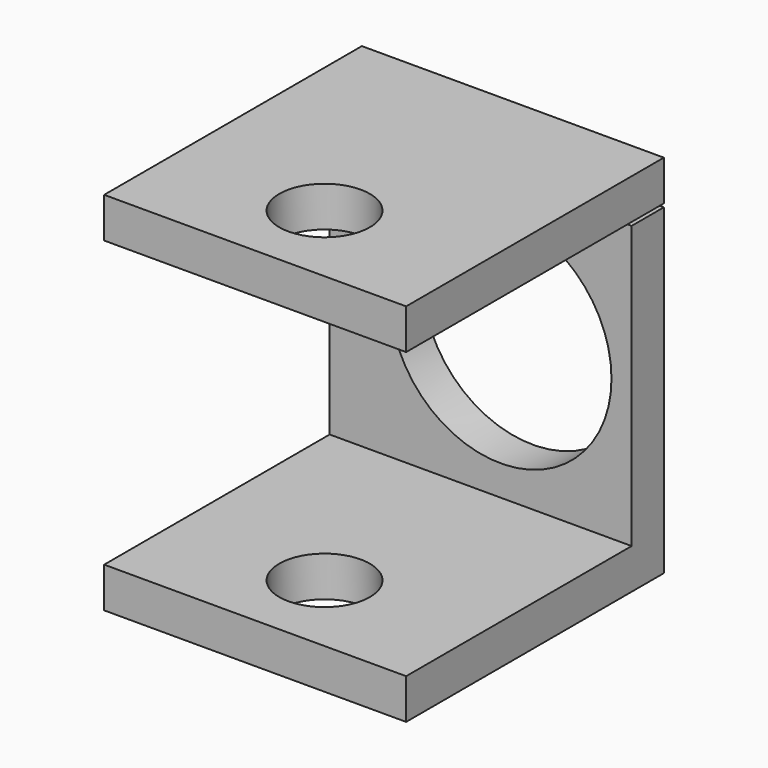
from build123d import *

# Parameters (mm, degrees)
F0_W     = 20.6375
F0_H     = 22.225
F0_R     = 8.73125
F1_DEPTH = 3.175
F2_DEPTH = 25.4
F4_D     = 7.14375


# Not quite as in the source:
# - a length typed as a fraction of an inch, garbled in the dataset ("3 / 203.2 mm" for 3/8 in), is restored


with BuildPart() as f1:
    # F0 (on Front) → F1 (new body)
    with BuildSketch(Plane.XZ):
        Rectangle(F0_W, F0_H)
        Circle(F0_R, mode=Mode.SUBTRACT)
        Polygon((-10.31875, -11.1125), (-10.31875, 11.1125), (-10.31875, 11.3854380324), (-13.49375, 11.3854380324), (-13.49375, -11.1125), align=None)
    extrude(amount=F1_DEPTH)

    # F0 (on Front) → F2 (join)
    with BuildSketch(Plane.XZ):
        Polygon((10.31875, -14.2875), (10.31875, -11.1125), (-10.31875, -11.1125), (-13.49375, -11.1125), (-13.49375, -14.2875), align=None)
        Polygon((-13.49375, 11.3854380324), (-10.31875, 11.3854380324), (10.31875, 11.3854380324), (10.31875, 14.5604380324), (-13.49375, 14.5604380324), align=None)
    extrude(amount=F2_DEPTH)

    # F4 (through all)
    with Locations(Plane(origin=(0, 0, -14.2875), x_dir=(1, 0, 0), z_dir=(0, 0, -1))):
        with Locations((-1.5875, 18.5598246753)):
            Hole(F4_D / 2)


solid = f1.part
